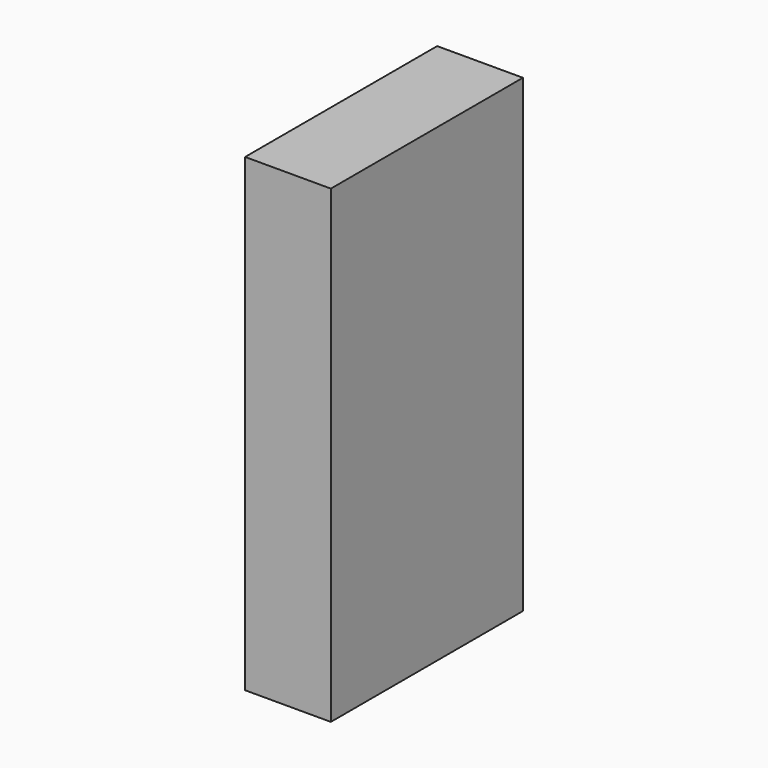
from build123d import *

# Parameters (mm, degrees)
F1_DEPTH = 1


# Not quite as in the source:
# - a feature names something its author has since deleted; it is built from what else it names


with BuildPart() as f1:
    # F0 (on Right) → F1 (new body)
    with BuildSketch(Plane.YZ):
        Polygon((4.35, -25), (5.25, -25), (6.25, -25), (7.15, -25), (7.15, -19.52432096), (4.35, -19.52432096), align=None)
    extrude(amount=F1_DEPTH)


solid = f1.part
